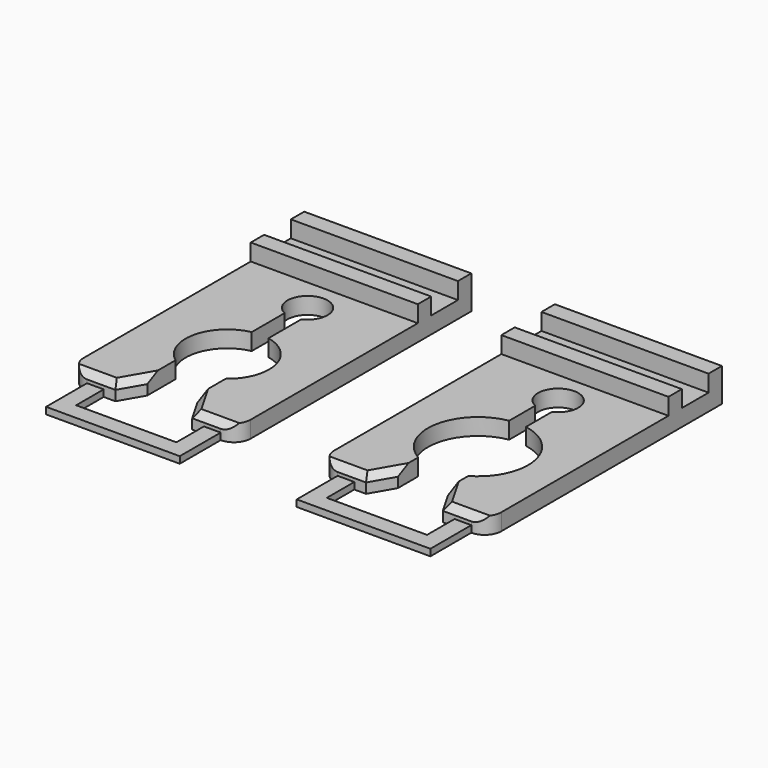
from build123d import *

# Parameters (mm, degrees)
F0_W        = 10
F0_H        = 1
F0_H_2      = 2
F1_DEPTH    = 1
F2_DEPTH    = 2
F3_R        = 1
F4_SIZE2    = 1.3856406461
F4_SIZE     = 0.8
F5_SIZE2    = 1.3856406461
F5_SIZE     = 0.8
F6_T1_DEPTH = 3.7573463904
F6_T3_DEPTH = 3.7573463904
F6_T5_DEPTH = 3.6573463904
F6_T7_DEPTH = 3.6573463904
F0_W_2      = 1
F0_H_3      = 2.0591422394
F7_DEPTH    = 0.4
F10_DEPTH   = 2


# Not quite as in the source:
# - a fillet or chamfer that OpenCascade refuses, or shapes differently, is made with other operations: its cross-section is extruded or revolved along the edge and cut away or added


with BuildPart() as f1:
    # F0 (on Top) → F1 (new body)
    with BuildSketch(Plane.XY):
        with Locations((0, 11.5)):
            Rectangle(F0_W, F0_H)
        with Locations((0, 10)):
            Rectangle(F0_W, F0_H_2)
        with Locations((0, 8.5)):
            Rectangle(F0_W, F0_H)
        with BuildLine():
            ThreePointArc((0.5, 2.4494897428), (1.9364916731, 1.5811388301), (2.5, 0))
            ThreePointArc((2.5, 0), (2.2360679775, -1.1180339887), (1.5, -2))
            Line((1.5, -2), (1.5, -5.5))
            Line((1.5, -5.5), (3, -5.5))
            Line((3, -5.5), (4, -5.5))
            Line((4, -5.5), (5, -5.5))
            Line((5, -5.5), (5, 8))
            Line((5, 8), (-5, 8))
            Line((-5, 8), (-5, -5.5))
            Line((-5, -5.5), (-4, -5.5))
            Line((-4, -5.5), (-3, -5.5))
            Line((-3, -5.5), (-1.5, -5.5))
            Line((-1.5, -5.5), (-1.5, -2))
            ThreePointArc((-1.5, -2), (-2.4391575888, 0.5481881586), (-0.5, 2.4494897428))
            Line((-0.5, 2.4494897428), (-0.5, 4.9091287885))
            ThreePointArc((-0.5, 4.9091287885), (-0.6480740698, 7.0099504938), (1.2, 6))
            ThreePointArc((1.2, 6), (1.0099504938, 5.3519259302), (0.5, 4.9091287885))
            Line((0.5, 4.9091287885), (0.5, 2.4494897428))
        make_face()
    extrude(amount=F1_DEPTH)

    # F0 (on Top) → F2 (join)
    with BuildSketch(Plane.XY):
        with Locations((0, 11.5)):
            Rectangle(F0_W, F0_H)
        with Locations((0, 8.5)):
            Rectangle(F0_W, F0_H)
    extrude(amount=F2_DEPTH)

    # F3
    f3_edges = [f1.edges().sort_by_distance(p)[0] for p in [
        (-5, -5.5, 0.5),
        (5, -5.5, 0.5),
    ]]
    fillet(f3_edges, radius=F3_R)

    # F4
    f4_edges = [f1.edges().sort_by_distance(p)[0] for p in [
        (-1.5, -5.5, 0.5),
    ]]
    f4_side = f1.faces().sort_by_distance((-2.75, -5.5, 0.5))[0]
    chamfer(f4_edges, length=F4_SIZE, length2=F4_SIZE2, reference=f4_side)

    # F5
    f5_edges = [f1.edges().sort_by_distance(p)[0] for p in [
        (1.5, -5.5, 0.5),
    ]]
    f5_side = f1.faces().sort_by_distance((2.75, -5.5, 0.5))[0]
    chamfer(f5_edges, length=F5_SIZE, length2=F5_SIZE2, reference=f5_side)

    # F6: chamfer of 0.4 on 4 edges, made by hand

    # F6_s2 → F6_t1 (cut)
    with BuildSketch(Plane.YZ.offset(-5.0286731952)):
        Polygon((-5.5, 0.6), (-5.1, 1), (-5.5, 1), align=None)
    extrude(amount=F6_T1_DEPTH, mode=Mode.SUBTRACT)

    # F6_s4 → F6_t3 (cut)
    with BuildSketch(Plane.YZ.offset(1.2713268048)):
        Polygon((-5.5, 0.6), (-5.1, 1), (-5.5, 1), align=None)
    extrude(amount=F6_T3_DEPTH, mode=Mode.SUBTRACT)

    # F6_s6 → F6_t5 (cut)
    with BuildSketch(Plane(origin=(-3.470906458, -6.0117863336, 0), x_dir=(0, 0, 1), z_dir=(0.5, 0.8660254038, 0))):
        Polygon((0.6, 0.7581415713), (1, 0.3581415713), (1, 0.7581415713), align=None)
    extrude(amount=F6_T5_DEPTH, mode=Mode.SUBTRACT)

    # F6_s8 → F6_t7 (cut)
    with BuildSketch(Plane(origin=(3.470906458, -6.0117863336, 0), x_dir=(0, 0, 1), z_dir=(-0.5, 0.8660254038, 0))):
        Polygon((0.6, -0.7581415713), (1, -0.3581415713), (1, -0.7581415713), align=None)
    extrude(amount=F6_T7_DEPTH, mode=Mode.SUBTRACT)

    # F0 (on Top) → F7 (join)
    with BuildSketch(Plane.XY):
        with Locations((-3.5, -6.5295711197)):
            Rectangle(F0_W_2, F0_H_3)
        Polygon((4, -7.5591422394), (3, -7.5591422394), (-3, -7.5591422394), (-4, -7.5591422394), (-4, -8.5591422394), (4, -8.5591422394), align=None)
        with Locations((3.5, -6.5295711197)):
            Rectangle(F0_W_2, F0_H_3)
    extrude(amount=F7_DEPTH)


with BuildPart() as f8_1:
    # F8: copy of F1
    add(f1.part.moved(Location((15, 0, 0))))

    # F9 (on face) → F10 (cut)
    with BuildSketch(Plane(origin=(0, 0, 0), x_dir=(1, 0, 0), z_dir=(0, 0, -1))):
        with BuildLine():
            ThreePointArc((15.5, -2.9580398915), (17.2912878475, -1.9364916731), (18, 0))
            ThreePointArc((18, 0), (17.5980762114, 1.5), (16.5, 2.5980762114))
            Line((16.5, 2.5980762114), (16.5, 2))
            ThreePointArc((16.5, 2), (17.4391575888, -0.5481881586), (15.5, -2.4494897428))
            Line((15.5, -2.4494897428), (15.5, -2.9580398915))
        make_face()
        with BuildLine():
            Line((13.5, 2), (13.5, 2.5980762114))
            ThreePointArc((13.5, 2.5980762114), (12.0474406801, -0.5314070594), (14.5, -2.9580398915))
            Line((14.5, -2.9580398915), (14.5, -2.4494897428))
            ThreePointArc((14.5, -2.4494897428), (12.5608424112, -0.5481881586), (13.5, 2))
        make_face()
    extrude(amount=-F10_DEPTH, mode=Mode.SUBTRACT)


solid = Compound([f1.part, f8_1.part])
